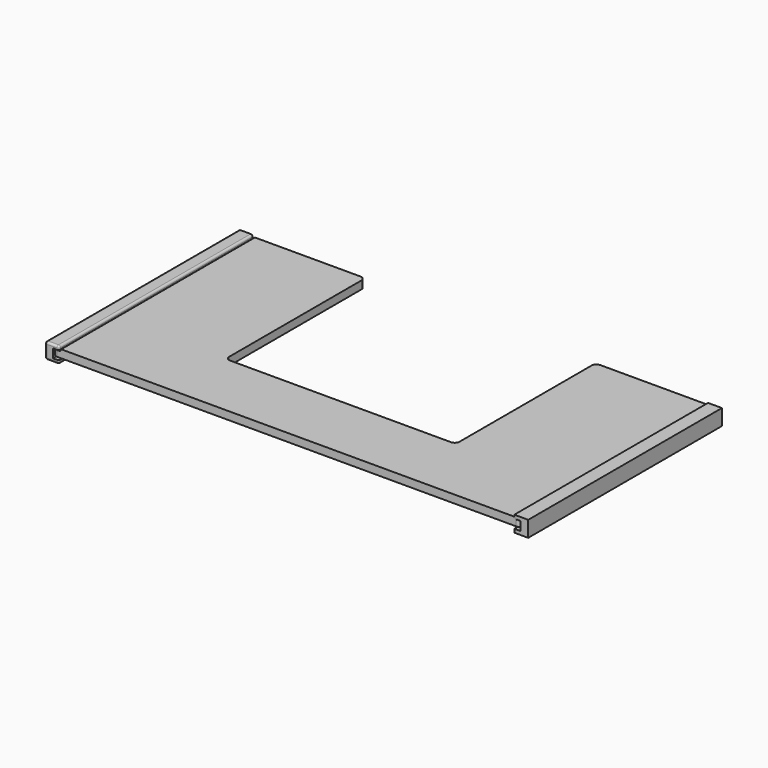
from build123d import *

# Parameters (mm, degrees)
F0_W      = 749.3
F0_H      = 12.7
F1_DEPTH  = 193.675
F2_W      = 368.3
F2_H      = 279.4
F3_DEPTH  = 12.7
F4_R      = 7.62
F6_DEPTH  = 3.175
F9_W      = 9.525
F9_H      = 387.35
F10_DEPTH = 3.175
F12_DEPTH = 387.35
F14_DEPTH = 387.35
F16_R     = 3.17499
F16_2_R   = 3.17499
F16_3_R   = 3.17499


# Not quite as in the source:
# - a fillet or chamfer is up to 0.001 mm smaller than in the source, because OpenCascade refuses the exact size
# - a feature of the source that left no trace in its solid (it failed there, or was rolled back) is left out
# - a pattern or mirror of a feature is missing from the dataset's text; its kind, count and spacing are read off the source's solid


with BuildPart() as f1:
    # F0 (on Front) → F1 (new body, symmetric)
    with BuildSketch(Plane.XZ):
        Rectangle(F0_W, F0_H)
    extrude(amount=F1_DEPTH, both=True)

    # F2 (on face) → F3 (cut, symmetric)
    with BuildSketch(Plane.XY.offset(6.35)):
        with Locations((0, 53.975)):
            Rectangle(F2_W, F2_H)
    extrude(amount=F3_DEPTH, both=True, mode=Mode.SUBTRACT)

    # F4
    f4_edges = [f1.edges().sort_by_distance(p)[0] for p in [
        (-184.15, 193.675, 0),
        (-374.65, 193.675, 0),
        (-184.15, -85.725, 0),
        (184.15, -85.725, 0),
        (184.15, 193.675, 0),
        (374.65, 193.675, 0),
        (374.65, -193.675, 0),
        (-374.65, -193.675, 0),
    ]]
    fillet(f4_edges, radius=F4_R)

    # F5 (on face) → F6 (cut)
    with BuildSketch(Plane.XY.offset(6.35)):
        with BuildLine():
            Line((-360.706291008, -193.675), (-360.706291008, 193.675))
            Line((-360.706291008, 193.675), (-368.3, 193.675))
            ThreePointArc((-368.3, 193.675), (-372.7901280605, 191.8151280605), (-374.65, 187.325))
            Line((-374.65, 187.325), (-374.65, -193.675))
            Line((-374.65, -193.675), (-360.706291008, -193.675))
        make_face()
    extrude(amount=-F6_DEPTH, mode=Mode.SUBTRACT)

    # F9 (on face) → F10 (cut)
    with BuildSketch(Plane.XY.offset(6.35)):
        with Locations((369.8875, 0)):
            Rectangle(F9_W, F9_H)
    extrude(amount=-F10_DEPTH, mode=Mode.SUBTRACT)

    # F11 (on face) → F12 (join)
    with BuildSketch(Plane.XZ.offset(193.675)):
        with BuildLine():
            ThreePointArc((368.3, 3.175), (366.0549359697, 4.1049359697), (365.125, 6.35))
            Line((365.125, 6.35), (365.125, 3.175))
            Line((365.125, 3.175), (368.3, 3.175))
        make_face()
    extrude(amount=-F12_DEPTH)


with BuildPart() as f14:
    # F13 (on face) → F14 (new body)
    with BuildSketch(Plane.XZ.offset(193.675)):
        Polygon((-364.262291008, 3.556), (-364.262291008, 9.144), (-386.487291008, 9.144), (-386.487291008, -16.256), (-364.262291008, -16.256), (-364.262291008, -10.668), (-373.787291008, -10.668), (-373.787291008, 3.556), align=None)
    extrude(amount=-F14_DEPTH)


with BuildPart() as f14_copies_1:
    # F14_copies: instance of F14
    add(f14.part.mirror(Plane(origin=(0, 0, 0), x_dir=(0, 0, 1), z_dir=(1, 0, 0))))


with BuildPart() as f15_1:
    # F15: copy of F1
    add(f1.part)

    # F16#3 (radius 3.175 in the source; OpenCascade refuses exactly that, so slightly less here)
    f16_3_edges = [f15_1.edges().sort_by_distance(p)[0] for p in [
        (-360.706291, 0, 3.175),
    ]]
    fillet(f16_3_edges, radius=F16_3_R)


with BuildPart() as f14_1:
    add(f14.part)

    # F16 (radius 3.175 in the source; OpenCascade refuses exactly that, so slightly less here)
    f16_edges = [f14_1.edges().sort_by_distance(p)[0] for p in [
        (-386.487291, 0, 9.144),
        (-375.374791, -193.675, 9.144),
        (-386.487291, -193.675, -3.556),
        (-386.487291, 0, -16.256),
        (-375.374791, -193.675, -16.256),
        (-364.262291, -193.675, -13.462),
        (-364.262291, -193.675, 6.35),
        (-364.262291, 0, 9.144),
        (-364.262291, 0, -16.256),
    ]]
    fillet(f16_edges, radius=F16_R)


with BuildPart() as f1_1:
    add(f1.part)

    # F16#2 (radius 3.175 in the source; OpenCascade refuses exactly that, so slightly less here)
    f16_2_edges = [f1_1.edges().sort_by_distance(p)[0] for p in [
        (-360.706291, 0, 3.175),
    ]]
    fillet(f16_2_edges, radius=F16_2_R)


solid = Compound([f14_copies_1.part, f15_1.part, f14_1.part, f1_1.part])
